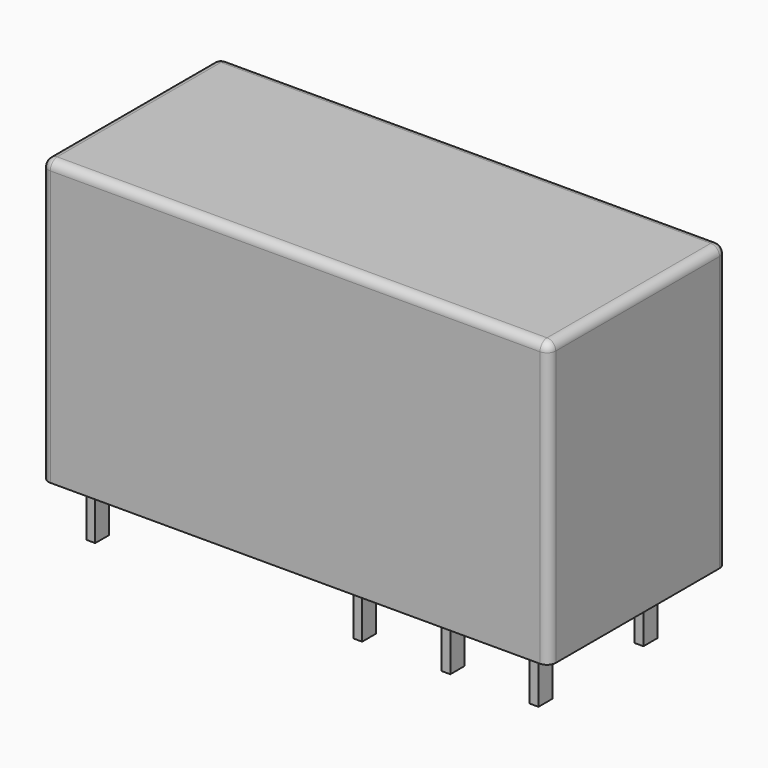
from build123d import *

# Parameters (mm, degrees)
F0_W     = 29
F0_H     = 16.2
F1_DEPTH = 12.7
F2_W     = 0.5
F2_H     = 1
F3_DEPTH = 3.6
F4_R     = 0.5


# Not quite as in the source:
# - a feature names something its author has since deleted; it is built from what else it names


with BuildPart() as f1:
    # F0 (on Front) → F1 (new body)
    with BuildSketch(Plane.XZ):
        Rectangle(F0_W, F0_H)
    extrude(amount=F1_DEPTH)

    # F4
    f4_edges = [f1.edges().sort_by_distance(p)[0] for p in [
        (-14.5, -12.7, 0),
        (0, -12.7, 8.1),
        (-14.5, -6.35, 8.1),
        (0, 0, 8.1),
        (14.5, -6.35, 8.1),
        (14.5, -12.7, 0),
        (14.5, 0, 0),
        (-14.5, 0, 0),
    ]]
    fillet(f4_edges, radius=F4_R)


with BuildPart() as f3:
    # F2 (on face) → F3 (new body)
    with BuildSketch(Plane(origin=(0, 0, -8.1), x_dir=(1, 0, 0), z_dir=(0, 0, -1))):
        with Locations((1.9, 2.6)):
            Rectangle(F2_W, F2_H)
    extrude(amount=F3_DEPTH)


with BuildPart() as f3b:
    # F2 (on face) → F3, piece 2 (new body)
    with BuildSketch(Plane(origin=(0, 0, -8.1), x_dir=(1, 0, 0), z_dir=(0, 0, -1))):
        with Locations((1.9, 10.1)):
            Rectangle(F2_W, F2_H)
    extrude(amount=F3_DEPTH)


with BuildPart() as f3c:
    # F2 (on face) → F3, piece 3 (new body)
    with BuildSketch(Plane(origin=(0, 0, -8.1), x_dir=(1, 0, 0), z_dir=(0, 0, -1))):
        with Locations((6.94, 10.1)):
            Rectangle(F2_W, F2_H)
    extrude(amount=F3_DEPTH)


with BuildPart() as f3d:
    # F2 (on face) → F3, piece 4 (new body)
    with BuildSketch(Plane(origin=(0, 0, -8.1), x_dir=(1, 0, 0), z_dir=(0, 0, -1))):
        with Locations((11.98, 10.1)):
            Rectangle(F2_W, F2_H)
    extrude(amount=F3_DEPTH)


with BuildPart() as f3e:
    # F2 (on face) → F3, piece 5 (new body)
    with BuildSketch(Plane(origin=(0, 0, -8.1), x_dir=(1, 0, 0), z_dir=(0, 0, -1))):
        with Locations((6.94, 2.6)):
            Rectangle(F2_W, F2_H)
    extrude(amount=F3_DEPTH)


with BuildPart() as f3f:
    # F2 (on face) → F3, piece 6 (new body)
    with BuildSketch(Plane(origin=(0, 0, -8.1), x_dir=(1, 0, 0), z_dir=(0, 0, -1))):
        with Locations((11.98, 2.6)):
            Rectangle(F2_W, F2_H)
    extrude(amount=F3_DEPTH)


with BuildPart() as f3g:
    # F2 (on face) → F3, piece 7 (new body)
    with BuildSketch(Plane(origin=(0, 0, -8.1), x_dir=(1, 0, 0), z_dir=(0, 0, -1))):
        with Locations((-13.36, 10.1)):
            Rectangle(F2_W, F2_H)
    extrude(amount=F3_DEPTH)


with BuildPart() as f3h:
    # F2 (on face) → F3, piece 8 (new body)
    with BuildSketch(Plane(origin=(0, 0, -8.1), x_dir=(1, 0, 0), z_dir=(0, 0, -1))):
        with Locations((-13.36, 2.6)):
            Rectangle(F2_W, F2_H)
    extrude(amount=F3_DEPTH)


solid = Compound([f1.part, f3.part, f3b.part, f3c.part, f3d.part, f3e.part, f3f.part, f3g.part, f3h.part])
